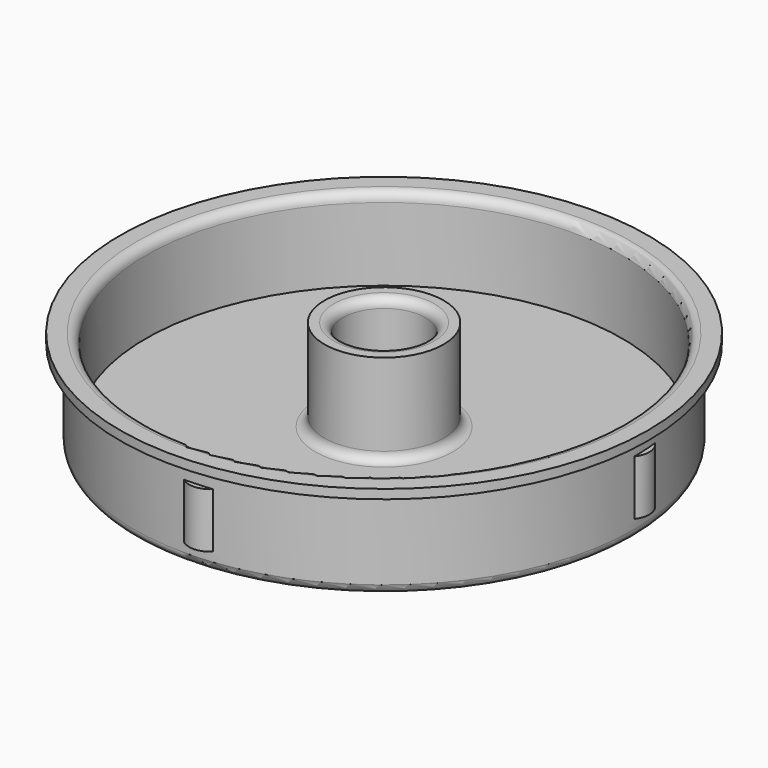
from build123d import *

# Parameters (mm, degrees)
F0_R      = 27.3
F0_R_2    = 4.5
F1_DEPTH  = 10
F2_R      = 26
F2_R_2    = 6.5
F3_DEPTH  = 8
F4_R      = 28.8
F4_R_2    = 27.3
F4_R_3    = 26
F5_DEPTH  = 1
F6_R      = 6.5
F6_R_2    = 4.5
F7_DEPTH  = 2
F8_R      = 0.99999
F8_2_R    = 0.99999
F10_START = -2
F10_DEPTH = 6
F11_R     = 1


# Not quite as in the source:
# - a fillet or chamfer is up to 0.001 mm smaller than in the source, because OpenCascade refuses the exact size


with BuildPart() as f1:
    # F0 (on Top) → F1 (new body)
    with BuildSketch(Plane.XY):
        Circle(F0_R)
        Circle(F0_R_2, mode=Mode.SUBTRACT)
    extrude(amount=F1_DEPTH)

    # F2 (on face) → F3 (cut)
    with BuildSketch(Plane.XY.offset(10)):
        Circle(F2_R)
        Circle(F2_R_2, mode=Mode.SUBTRACT)
    extrude(amount=-F3_DEPTH, mode=Mode.SUBTRACT)

    # F6 (on face) → F7 (join)
    with BuildSketch(Plane.XY.offset(10)):
        Circle(F6_R)
        Circle(F6_R_2, mode=Mode.SUBTRACT)
    extrude(amount=F7_DEPTH)

    # F8 (radius 1 in the source; OpenCascade refuses exactly that, so slightly less here)
    f8_edges = [f1.edges().sort_by_distance(p)[0] for p in [
        (-4.5, 0, 0),
        (-4.5, 0, 12),
        (-6.5, 0, 2),
    ]]
    fillet(f8_edges, radius=F8_R)

    # F9 (on face) → F10 (join)
    with BuildSketch(Plane(origin=(0, 0, 0), x_dir=(1, 0, 0), z_dir=(0, 0, -1)).offset(F10_START)):
        with BuildLine():
            ThreePointArc((27.1294434502, -3.0468505187), (27.7866214105, -1.5554390509), (27.3, 0))
            ThreePointArc((27.3, 0), (27.257327512, -1.5258102454), (27.1294434502, -3.0468505187))
        make_face()
        with BuildLine():
            ThreePointArc((-27.3, 0), (-27.257327512, 1.5258102454), (-27.1294434502, 3.0468505187))
            ThreePointArc((-27.1294434502, 3.0468505187), (-27.7866214105, 1.5554390509), (-27.3, 0))
        make_face()
        with BuildLine():
            ThreePointArc((3.0468505187, 27.1294434502), (1.5554390509, 27.7866214105), (0, 27.3))
            ThreePointArc((0, 27.3), (1.5258102454, 27.257327512), (3.0468505187, 27.1294434502))
        make_face()
        with BuildLine():
            ThreePointArc((0, -27.3), (-1.5258102454, -27.257327512), (-3.0468505187, -27.1294434502))
            ThreePointArc((-3.0468505187, -27.1294434502), (-1.5554390509, -27.7866214105), (0, -27.3))
        make_face()
    extrude(amount=-F10_DEPTH)

    # F11
    f11_edges = [f1.edges().sort_by_distance(p)[0] for p in [
        (-27.3, 0, 0),
    ]]
    fillet(f11_edges, radius=F11_R)


with BuildPart() as f5:
    # F4 (on face) → F5 (new body)
    with BuildSketch(Plane.XY.offset(10)):
        Circle(F4_R)
        Circle(F4_R_2, mode=Mode.SUBTRACT)
        Circle(F4_R_2)
        Circle(F4_R_3, mode=Mode.SUBTRACT)
    extrude(amount=F5_DEPTH)

    # F8#2 (radius 1 in the source; OpenCascade refuses exactly that, so slightly less here)
    f8_2_edges = [f5.edges().sort_by_distance(p)[0] for p in [
        (-26, 0, 11),
    ]]
    fillet(f8_2_edges, radius=F8_2_R)


solid = Compound([f1.part, f5.part])
